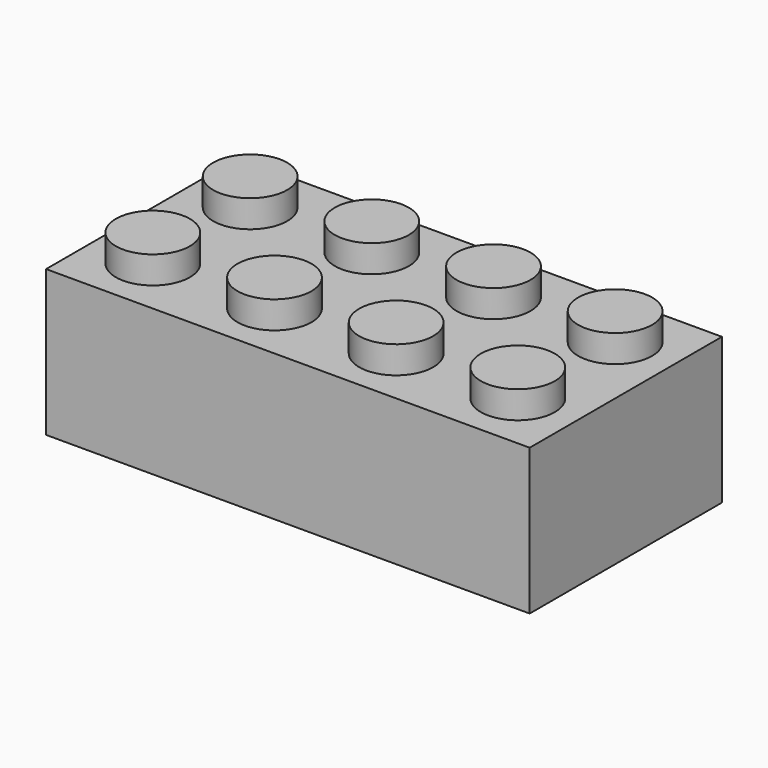
from build123d import *

# Parameters (mm, degrees)
F0_W        = 31.8
F0_H        = 15.8
F1_DEPTH    = 9.6
F2_R        = 2.435
F3_DEPTH    = 1.8
F4_T        = -1.24
F5_R        = 3.2
F6_DEPTH    = 8.36
F7_T        = 1.24
F7_T3_DEPTH = 10.84
F7_T5_DEPTH = 15.8
F7_T7_DEPTH = 31.8
F9_DEPTH    = 5


# Not quite as in the source:
# - a shell that OpenCascade refuses in one call is made with other operations: the cavity is built on its own and cut out


with BuildPart() as f1:
    # F0 (on Top) → F1 (new body)
    with BuildSketch(Plane.XY):
        with Locations((15.9, 7.9)):
            Rectangle(F0_W, F0_H)
    extrude(amount=F1_DEPTH)

    # F2 (on face) → F3 (join)
    with BuildSketch(Plane.XY.offset(9.6)):
        with Locations((11.9, 11.9)):
            Circle(F2_R)
        with Locations((19.9, 11.9)):
            Circle(F2_R)
        with Locations((27.9, 11.9)):
            Circle(F2_R)
        with Locations((27.9, 3.9)):
            Circle(F2_R)
        with Locations((19.9, 3.9)):
            Circle(F2_R)
        with Locations((11.9, 3.9)):
            Circle(F2_R)
        with Locations((3.9, 3.9)):
            Circle(F2_R)
        with Locations((3.9, 11.9)):
            Circle(F2_R)
    extrude(amount=F3_DEPTH)

    # F4
    f4_openings = [f1.faces().sort_by_distance(p)[0] for p in [
        (15.9, 7.9, 0),
    ]]
    offset(amount=F4_T, openings=f4_openings, kind=Kind.INTERSECTION)

    # F5 (on face) → F6 (join, through all)
    with BuildSketch(Plane(origin=(0, 0, 8.36), x_dir=(1, 0, 0), z_dir=(0, 0, -1))):
        with Locations((7.9, -7.9)):
            Circle(F5_R)
        with Locations((15.9, -7.9)):
            Circle(F5_R)
        with Locations((23.9, -7.9)):
            Circle(F5_R)
    extrude(amount=F6_DEPTH)

    # F7: shell of thickness 1.24, made by hand


with BuildPart() as f7_core1:
    # F7_t2: copy of F1
    add(f1.part)

    # the walls: a layer under each face that stays
    f7_faces = [f7_core1.faces().sort_by_distance(p)[0] for p in [
        (0, 7.9, 4.8),
        (15.9, 15.8, 4.8),
        (15.9, 0, 4.8),
        (2.2714285714, 1.1285714286, 0),
        (15.9, 7.9, 9.6),
        (31.8, 7.9, 4.8),
        (1.24, 7.9, 4.18),
        (15.9, 14.56, 4.18),
        (30.56, 7.9, 4.18),
        (15.9, 1.24, 4.18),
        (1.465, 3.9, 10.5),
        (9.465, 3.9, 10.5),
        (17.465, 3.9, 10.5),
        (25.465, 3.9, 10.5),
        (1.465, 11.9, 10.5),
        (9.465, 11.9, 10.5),
        (17.465, 11.9, 10.5),
        (25.465, 11.9, 10.5),
        (6.1266666667, 3.46, 8.36),
        (3.9, 3.9, 11.4),
        (11.9, 3.9, 11.4),
        (19.9, 3.9, 11.4),
        (27.9, 3.9, 11.4),
        (3.9, 11.9, 11.4),
        (11.9, 11.9, 11.4),
        (19.9, 11.9, 11.4),
        (27.9, 11.9, 11.4),
        (2.705, 3.9, 9.26),
        (10.705, 3.9, 9.26),
        (18.705, 3.9, 9.26),
        (26.705, 3.9, 9.26),
        (4.7, 7.9, 4.18),
        (2.705, 11.9, 9.26),
        (10.705, 11.9, 9.26),
        (12.7, 7.9, 4.18),
        (20.7, 7.9, 4.18),
        (18.705, 11.9, 9.26),
        (26.705, 11.9, 9.26),
        (3.9, 3.9, 10.16),
        (11.9, 3.9, 10.16),
        (19.9, 3.9, 10.16),
        (27.9, 3.9, 10.16),
        (3.9, 11.9, 10.16),
        (11.9, 11.9, 10.16),
        (19.9, 11.9, 10.16),
        (27.9, 11.9, 10.16),
    ]]
    thicken(f7_faces, amount=-F7_T, mode=Mode.SUBTRACT)

    # F7_s4 → F7_t3 (cut)
    with BuildSketch(Plane.XY.offset(-1.24)):
        Polygon((1.2524, 14.5476), (0, 14.56), (0, 15.8), (1.24, 15.8), align=None)
        Polygon((1.2524, 1.2524), (0, 1.24), (0, 0), (1.24, 0), align=None)
        Polygon((30.5476, 14.5476), (30.56, 15.8), (31.8, 15.8), (31.8, 14.56), align=None)
        Polygon((30.5476, 1.2524), (31.8, 1.24), (31.8, 0), (30.56, 0), align=None)
    extrude(amount=F7_T3_DEPTH, mode=Mode.SUBTRACT)

    # F7_s6 → F7_t5 (cut)
    with BuildSketch(Plane.XZ.offset(-15.8)):
        Polygon((1.2524, 8.3476), (0, 8.36), (0, 9.6), (1.24, 9.6), align=None)
        Polygon((30.5476, 8.3476), (31.8, 8.36), (31.8, 9.6), (30.56, 9.6), align=None)
    extrude(amount=F7_T5_DEPTH, mode=Mode.SUBTRACT)

    # F7_s8 → F7_t7 (cut)
    with BuildSketch(Plane.YZ):
        Polygon((14.5476, 8.3476), (15.8, 8.36), (15.8, 9.6), (14.56, 9.6), align=None)
        Polygon((1.2524, 8.3476), (0, 8.36), (0, 9.6), (1.24, 9.6), align=None)
    extrude(amount=F7_T7_DEPTH, mode=Mode.SUBTRACT)

    # F7_s9 → F7_t10 (revolve, cut)
    with BuildSketch(Plane.XZ.offset(-3.9)):
        Polygon((6.3474, 9.6124), (6.335, 8.36), (5.095, 8.36), (5.095, 9.6), align=None)
    revolve(axis=Axis((3.9, 3.9, 9.6), (0, 0, 1)), mode=Mode.SUBTRACT)

    # F7_s11 → F7_t12 (revolve, cut)
    with BuildSketch(Plane.XZ.offset(-3.9)):
        Polygon((14.3474, 9.6124), (14.335, 8.36), (13.095, 8.36), (13.095, 9.6), align=None)
    revolve(axis=Axis((11.9, 3.9, 9.6), (0, 0, 1)), mode=Mode.SUBTRACT)

    # F7_s13 → F7_t14 (revolve, cut)
    with BuildSketch(Plane.XZ.offset(-3.9)):
        Polygon((22.3474, 9.6124), (22.335, 8.36), (21.095, 8.36), (21.095, 9.6), align=None)
    revolve(axis=Axis((19.9, 3.9, 9.6), (0, 0, 1)), mode=Mode.SUBTRACT)

    # F7_s15 → F7_t16 (revolve, cut)
    with BuildSketch(Plane.XZ.offset(-3.9)):
        Polygon((30.3474, 9.6124), (30.335, 8.36), (29.095, 8.36), (29.095, 9.6), align=None)
    revolve(axis=Axis((27.9, 3.9, 9.6), (0, 0, 1)), mode=Mode.SUBTRACT)

    # F7_s17 → F7_t18 (revolve, cut)
    with BuildSketch(Plane.XZ.offset(-11.9)):
        Polygon((6.3474, 9.6124), (6.335, 8.36), (5.095, 8.36), (5.095, 9.6), align=None)
    revolve(axis=Axis((3.9, 11.9, 9.6), (0, 0, 1)), mode=Mode.SUBTRACT)

    # F7_s19 → F7_t20 (revolve, cut)
    with BuildSketch(Plane.XZ.offset(-11.9)):
        Polygon((14.3474, 9.6124), (14.335, 8.36), (13.095, 8.36), (13.095, 9.6), align=None)
    revolve(axis=Axis((11.9, 11.9, 9.6), (0, 0, 1)), mode=Mode.SUBTRACT)

    # F7_s21 → F7_t22 (revolve, cut)
    with BuildSketch(Plane.XZ.offset(-11.9)):
        Polygon((22.3474, 9.6124), (22.335, 8.36), (21.095, 8.36), (21.095, 9.6), align=None)
    revolve(axis=Axis((19.9, 11.9, 9.6), (0, 0, 1)), mode=Mode.SUBTRACT)

    # F7_s23 → F7_t24 (revolve, cut)
    with BuildSketch(Plane.XZ.offset(-11.9)):
        Polygon((30.3474, 9.6124), (30.335, 8.36), (29.095, 8.36), (29.095, 9.6), align=None)
    revolve(axis=Axis((27.9, 11.9, 9.6), (0, 0, 1)), mode=Mode.SUBTRACT)

    # F7_s25 → F7_t26 (revolve, cut)
    with BuildSketch(Plane.XZ.offset(-7.9)):
        Polygon((11.1124, 8.3476), (11.1, 9.6), (9.86, 9.6), (9.86, 8.36), align=None)
    revolve(axis=Axis((7.9, 7.9, 8.36), (0, 0, -1)), mode=Mode.SUBTRACT)

    # F7_s27 → F7_t28 (revolve, cut)
    with BuildSketch(Plane.XZ.offset(-7.9)):
        Polygon((19.1124, 8.3476), (19.1, 9.6), (17.86, 9.6), (17.86, 8.36), align=None)
    revolve(axis=Axis((15.9, 7.9, 8.36), (0, 0, -1)), mode=Mode.SUBTRACT)

    # F7_s29 → F7_t30 (revolve, cut)
    with BuildSketch(Plane.XZ.offset(-7.9)):
        Polygon((27.1124, 8.3476), (27.1, 9.6), (25.86, 9.6), (25.86, 8.36), align=None)
    revolve(axis=Axis((23.9, 7.9, 8.36), (0, 0, -1)), mode=Mode.SUBTRACT)

    # F7_s31 → F7_t32 (revolve, cut)
    with BuildSketch(Plane.XZ.offset(-3.9)):
        Polygon((5.0826, 10.1476), (6.335, 10.16), (6.335, 11.4), (5.095, 11.4), align=None)
    revolve(axis=Axis((3.9, 3.9, 10.16), (0, 0, -1)), mode=Mode.SUBTRACT)

    # F7_s33 → F7_t34 (revolve, cut)
    with BuildSketch(Plane.XZ.offset(-3.9)):
        Polygon((13.0826, 10.1476), (14.335, 10.16), (14.335, 11.4), (13.095, 11.4), align=None)
    revolve(axis=Axis((11.9, 3.9, 10.16), (0, 0, -1)), mode=Mode.SUBTRACT)

    # F7_s35 → F7_t36 (revolve, cut)
    with BuildSketch(Plane.XZ.offset(-3.9)):
        Polygon((21.0826, 10.1476), (22.335, 10.16), (22.335, 11.4), (21.095, 11.4), align=None)
    revolve(axis=Axis((19.9, 3.9, 10.16), (0, 0, -1)), mode=Mode.SUBTRACT)

    # F7_s37 → F7_t38 (revolve, cut)
    with BuildSketch(Plane.XZ.offset(-3.9)):
        Polygon((29.0826, 10.1476), (30.335, 10.16), (30.335, 11.4), (29.095, 11.4), align=None)
    revolve(axis=Axis((27.9, 3.9, 10.16), (0, 0, -1)), mode=Mode.SUBTRACT)

    # F7_s39 → F7_t40 (revolve, cut)
    with BuildSketch(Plane.XZ.offset(-11.9)):
        Polygon((5.0826, 10.1476), (6.335, 10.16), (6.335, 11.4), (5.095, 11.4), align=None)
    revolve(axis=Axis((3.9, 11.9, 10.16), (0, 0, -1)), mode=Mode.SUBTRACT)

    # F7_s41 → F7_t42 (revolve, cut)
    with BuildSketch(Plane.XZ.offset(-11.9)):
        Polygon((13.0826, 10.1476), (14.335, 10.16), (14.335, 11.4), (13.095, 11.4), align=None)
    revolve(axis=Axis((11.9, 11.9, 10.16), (0, 0, -1)), mode=Mode.SUBTRACT)

    # F7_s43 → F7_t44 (revolve, cut)
    with BuildSketch(Plane.XZ.offset(-11.9)):
        Polygon((21.0826, 10.1476), (22.335, 10.16), (22.335, 11.4), (21.095, 11.4), align=None)
    revolve(axis=Axis((19.9, 11.9, 10.16), (0, 0, -1)), mode=Mode.SUBTRACT)

    # F7_s45 → F7_t46 (revolve, cut)
    with BuildSketch(Plane.XZ.offset(-11.9)):
        Polygon((29.0826, 10.1476), (30.335, 10.16), (30.335, 11.4), (29.095, 11.4), align=None)
    revolve(axis=Axis((27.9, 11.9, 10.16), (0, 0, -1)), mode=Mode.SUBTRACT)


with BuildPart() as f1_1:
    add(f1.part)

    # what is left inside the walls is the cavity
    f7_cavity = [f7_core1.part.solids().sort_by_distance(p)[0] for p in [
        (5.9524, 7.9, 2.786667),
        (13.9524, 7.9, 2.786667),
        (21.9524, 7.9, 2.786667),
    ]]
    add(f7_cavity, mode=Mode.SUBTRACT)

    # F8 (on face) → F9 (join)
    with BuildSketch(Plane(origin=(0, 0, 8.36), x_dir=(1, 0, 0), z_dir=(0, 0, -1))):
        with BuildLine():
            Line((16.4, -1.24), (15.4, -1.24))
            Line((15.4, -1.24), (15.4, -4.7393038741))
            ThreePointArc((15.4, -4.7393038741), (15.9, -4.7), (16.4, -4.7393038741))
            Line((16.4, -4.7393038741), (16.4, -1.24))
        make_face()
        with BuildLine():
            ThreePointArc((16.4, -11.0606961259), (15.9, -11.1), (15.4, -11.0606961259))
            Line((15.4, -11.0606961259), (15.4, -14.56))
            Line((15.4, -14.56), (16.4, -14.56))
            Line((16.4, -14.56), (16.4, -11.0606961259))
        make_face()
    extrude(amount=F9_DEPTH)


solid = f1_1.part
